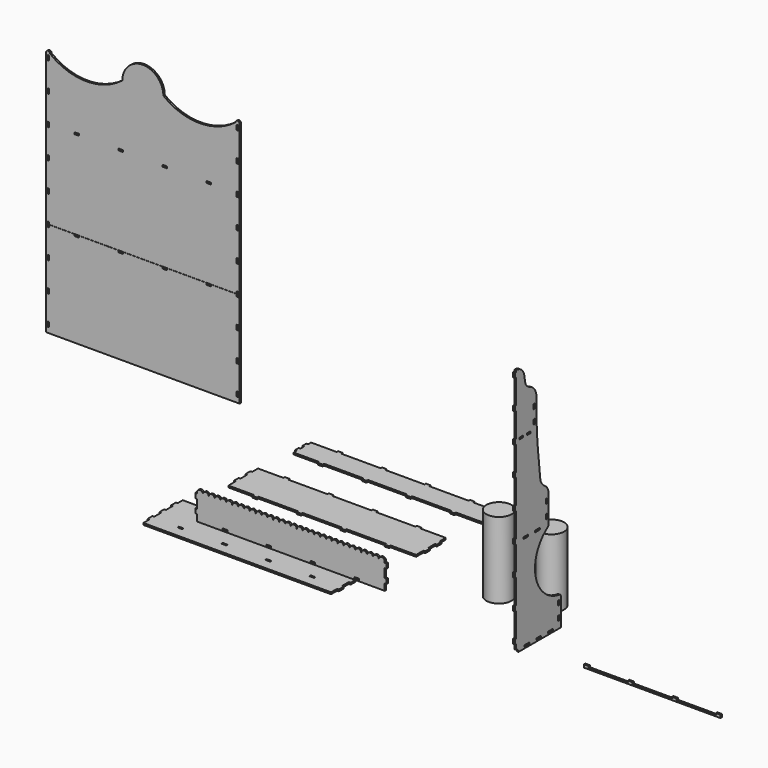
from build123d import *

# Parameters (mm, degrees)
F0_W      = 10
F0_H      = 3
F0_W_2    = 3
F0_H_2    = 8
F0_W_3    = 8
F1_DEPTH  = 3
F2_W      = 8
F2_H      = 3
F3_DEPTH  = 3
F4_W      = 8
F4_H      = 3
F5_DEPTH  = 3
F7_DEPTH  = 3
F9_DEPTH  = 3
F10_W     = 3
F10_H     = 8
F12_DEPTH = 3
F10_W_2   = 8
F10_H_2   = 3
F13_DEPTH = 3
F14_DEPTH = 3
F15_R     = 21.5
F16_DEPTH = 130
F17_DEPTH = 117


# Not quite as in the source:
# - a feature names something its author has since deleted; it is built from what else it names


with BuildPart() as f1:
    # F0 (on Right) → F1 (new body)
    with BuildSketch(Plane.YZ):
        with BuildLine():
            Line((0, 14), (0, 5))
            ThreePointArc((0, 5), (3.5355339059, 3.5355339059), (5, 0))
            Line((5, 0), (95, 0))
            Line((95, 0), (95, 47.3543956658))
            ThreePointArc((95, 47.3543956658), (94.2705921351, 49.3151127173), (92.4370590961, 50.3223881433))
            ThreePointArc((92.4370590961, 50.3223881433), (41.6413829378, 97.2032586539), (66.8184709068, 161.5781837226))
            ThreePointArc((66.8184709068, 161.5781837226), (68.4211058873, 163.372759507), (69, 165.7081016089))
            Line((69, 165.7081016089), (69, 213))
            ThreePointArc((69, 213), (66.3858613305, 220.9035210379), (60.5112875599, 226.8017198134))
            ThreePointArc((60.5112875599, 226.8017198134), (54.1229379519, 233.1545161459), (51.1709644901, 241.6665596512))
            Line((51.1709644901, 241.6665596512), (46.9762373129, 280.85384986))
            ThreePointArc((46.9762373129, 280.85384986), (45.2396853535, 299.4070999888), (43.9976015301, 318))
            ThreePointArc((43.9976015301, 318), (43.2494448273, 336.6725204464), (43, 355.3583582802))
            Line((43, 355.3583582802), (43, 369.5985722542))
            ThreePointArc((43, 369.5985722542), (38.5808045495, 380.9800883223), (28.6916338415, 388.1405700899))
            ThreePointArc((28.6916338415, 388.1405700899), (22.2280112249, 392.6087038732), (18.9101247071, 399.7315028939))
            Line((18.9101247071, 399.7315028939), (17.4928194431, 407.943180155))
            ThreePointArc((17.4928194431, 407.943180155), (12.2161147188, 420.0299862844), (0, 425))
            Line((0, 425), (0, 422))
            Line((0, 422), (-3, 422))
            Line((-3, 422), (-3, 414))
            Line((-3, 414), (0, 414))
            Line((0, 414), (0, 372))
            Line((0, 372), (-3, 372))
            Line((-3, 372), (-3, 364))
            Line((-3, 364), (0, 364))
            Line((0, 364), (0, 322))
            Line((0, 322), (-3, 322))
            Line((-3, 322), (-3, 314))
            Line((-3, 314), (0, 314))
            Line((0, 314), (0, 272))
            Line((0, 272), (-3, 272))
            Line((-3, 272), (-3, 264))
            Line((-3, 264), (0, 264))
            Line((0, 264), (0, 222))
            Line((0, 222), (-3, 222))
            Line((-3, 222), (-3, 214))
            Line((-3, 214), (0, 214))
            Line((0, 214), (0, 172))
            Line((0, 172), (-3, 172))
            Line((-3, 172), (-3, 164))
            Line((-3, 164), (0, 164))
            Line((0, 164), (0, 122))
            Line((0, 122), (-3, 122))
            Line((-3, 122), (-3, 114))
            Line((-3, 114), (0, 114))
            Line((0, 114), (0, 72))
            Line((0, 72), (-3, 72))
            Line((-3, 72), (-3, 64))
            Line((-3, 64), (0, 64))
            Line((0, 64), (0, 22))
            Line((0, 22), (-3, 22))
            Line((-3, 22), (-3, 14))
            Line((-3, 14), (0, 14))
        make_face()
        with Locations((23, 3.5)):
            Rectangle(F0_W, F0_H, mode=Mode.SUBTRACT)
        with Locations((20.5, 166.5)):
            Rectangle(F0_W, F0_H, mode=Mode.SUBTRACT)
        with Locations((45.5, 166.5)):
            Rectangle(F0_W, F0_H, mode=Mode.SUBTRACT)
        with Locations((48, 3.5)):
            Rectangle(F0_W, F0_H, mode=Mode.SUBTRACT)
        with Locations((73, 3.5)):
            Rectangle(F0_W, F0_H, mode=Mode.SUBTRACT)
        with Locations((90.5, 16)):
            Rectangle(F0_W_2, F0_H_2, mode=Mode.SUBTRACT)
        with Locations((90.5, 39)):
            Rectangle(F0_W_2, F0_H_2, mode=Mode.SUBTRACT)
        with Locations((64.5, 179)):
            Rectangle(F0_W_2, F0_H_2, mode=Mode.SUBTRACT)
        with Locations((64.5, 202)):
            Rectangle(F0_W_2, F0_H_2, mode=Mode.SUBTRACT)
        with Locations((10.5, 319.5)):
            Rectangle(F0_W_3, F0_H, mode=Mode.SUBTRACT)
        with Locations((26.5, 319.5)):
            Rectangle(F0_W_3, F0_H, mode=Mode.SUBTRACT)
        with Locations((38.5, 332)):
            Rectangle(F0_W_2, F0_H_2, mode=Mode.SUBTRACT)
        with Locations((38.5, 355)):
            Rectangle(F0_W_2, F0_H_2, mode=Mode.SUBTRACT)
    extrude(amount=F1_DEPTH)


with BuildPart() as f3:
    # F2 (on Top) → F3 (new body)
    with BuildSketch(Plane.XY):
        Polygon((-615.7709360123, -8.2306790054), (-615.7709360123, -21.2306790054), (-295.7709360123, -21.2306790054), (-295.7709360123, -8.2306790054), (-292.7709360123, -8.2306790054), (-292.7709360123, 1.7693209946), (-295.7709360123, 1.7693209946), (-295.7709360123, 16.7693209946), (-292.7709360123, 16.7693209946), (-292.7709360123, 26.7693209946), (-295.7709360123, 26.7693209946), (-295.7709360123, 41.7693209946), (-292.7709360123, 41.7693209946), (-292.7709360123, 51.7693209946), (-295.7709360123, 51.7693209946), (-295.7709360123, 62.7693209946), (-339.2709360123, 62.7693209946), (-339.2709360123, 65.7693209946), (-347.2709360123, 65.7693209946), (-347.2709360123, 62.7693209946), (-414.2709360123, 62.7693209946), (-414.2709360123, 65.7693209946), (-422.2709360123, 65.7693209946), (-422.2709360123, 62.7693209946), (-489.2709360123, 62.7693209946), (-489.2709360123, 65.7693209946), (-497.2709360123, 65.7693209946), (-497.2709360123, 62.7693209946), (-564.2709360123, 62.7693209946), (-564.2709360123, 65.7693209946), (-572.2709360123, 65.7693209946), (-572.2709360123, 62.7693209946), (-615.7709360123, 62.7693209946), (-615.7709360123, 51.7693209946), (-618.7709360123, 51.7693209946), (-618.7709360123, 41.7693209946), (-615.7709360123, 41.7693209946), (-615.7709360123, 26.7693209946), (-618.7709360123, 26.7693209946), (-618.7709360123, 16.7693209946), (-615.7709360123, 16.7693209946), (-615.7709360123, 1.7693209946), (-618.7709360123, 1.7693209946), (-618.7709360123, -8.2306790054), align=None)
        with Locations((-568.2709360123, -1.5)):
            Rectangle(F2_W, F2_H, mode=Mode.SUBTRACT)
        with Locations((-493.2709360123, -1.5)):
            Rectangle(F2_W, F2_H, mode=Mode.SUBTRACT)
        with Locations((-418.2709360123, -1.5)):
            Rectangle(F2_W, F2_H, mode=Mode.SUBTRACT)
        with Locations((-343.2709360123, -1.5)):
            Rectangle(F2_W, F2_H, mode=Mode.SUBTRACT)
    extrude(amount=F3_DEPTH)


with BuildPart() as f5:
    # F4 (on Front) → F5 (new body)
    with BuildSketch(Plane.XZ):
        with BuildLine():
            Line((-538.8287305832, 22.7397029996), (-218.8287305832, 22.7397029996))
            Line((-218.8287305832, 22.7397029996), (-218.8287305832, 33.7397029996))
            Line((-218.8287305832, 33.7397029996), (-215.8287305832, 33.7397029996))
            Line((-215.8287305832, 33.7397029996), (-215.8287305832, 41.7397029996))
            Line((-215.8287305832, 41.7397029996), (-218.8287305832, 41.7397029996))
            Line((-218.8287305832, 41.7397029996), (-218.8287305832, 56.7397029996))
            Line((-218.8287305832, 56.7397029996), (-215.8287305832, 56.7397029996))
            Line((-215.8287305832, 56.7397029996), (-215.8287305832, 64.7397029996))
            Line((-215.8287305832, 64.7397029996), (-218.8287305832, 64.7397029996))
            Line((-218.8287305832, 64.7397029996), (-218.8287305832, 66.7397029996))
            ThreePointArc((-218.8287305832, 66.7397029996), (-223.8287305832, 71.7397029996), (-228.8287305832, 66.7397029996))
            ThreePointArc((-228.8287305832, 66.7397029996), (-233.8287305832, 71.7397029996), (-238.8287305832, 66.7397029996))
            ThreePointArc((-238.8287305832, 66.7397029996), (-243.8287305832, 71.7397029996), (-248.8287305832, 66.7397029996))
            ThreePointArc((-248.8287305832, 66.7397029996), (-253.8287305832, 71.7397029996), (-258.8287305832, 66.7397029996))
            ThreePointArc((-258.8287305832, 66.7397029996), (-263.8287305832, 71.7397029996), (-268.8287305832, 66.7397029996))
            ThreePointArc((-268.8287305832, 66.7397029996), (-273.8287305832, 71.7397029996), (-278.8287305832, 66.7397029996))
            ThreePointArc((-278.8287305832, 66.7397029996), (-283.8287305832, 71.7397029996), (-288.8287305832, 66.7397029996))
            ThreePointArc((-288.8287305832, 66.7397029996), (-293.8287305832, 71.7397029996), (-298.8287305832, 66.7397029996))
            ThreePointArc((-298.8287305832, 66.7397029996), (-303.8287305832, 71.7397029996), (-308.8287305832, 66.7397029996))
            ThreePointArc((-308.8287305832, 66.7397029996), (-313.8287305832, 71.7397029996), (-318.8287305832, 66.7397029996))
            ThreePointArc((-318.8287305832, 66.7397029996), (-323.8287305832, 71.7397029996), (-328.8287305832, 66.7397029996))
            ThreePointArc((-328.8287305832, 66.7397029996), (-333.8287305832, 71.7397029996), (-338.8287305832, 66.7397029996))
            ThreePointArc((-338.8287305832, 66.7397029996), (-343.8287305832, 71.7397029996), (-348.8287305832, 66.7397029996))
            ThreePointArc((-348.8287305832, 66.7397029996), (-353.8287305832, 71.7397029996), (-358.8287305832, 66.7397029996))
            ThreePointArc((-358.8287305832, 66.7397029996), (-363.8287305832, 71.7397029996), (-368.8287305832, 66.7397029996))
            ThreePointArc((-368.8287305832, 66.7397029996), (-373.8287305832, 71.7397029996), (-378.8287305832, 66.7397029996))
            ThreePointArc((-378.8287305832, 66.7397029996), (-383.8287305832, 71.7397029996), (-388.8287305832, 66.7397029996))
            ThreePointArc((-388.8287305832, 66.7397029996), (-393.8287305832, 71.7397029996), (-398.8287305832, 66.7397029996))
            ThreePointArc((-398.8287305832, 66.7397029996), (-403.8287305832, 71.7397029996), (-408.8287305832, 66.7397029996))
            ThreePointArc((-408.8287305832, 66.7397029996), (-413.8287305832, 71.7397029996), (-418.8287305832, 66.7397029996))
            ThreePointArc((-418.8287305832, 66.7397029996), (-423.8287305832, 71.7397029996), (-428.8287305832, 66.7397029996))
            ThreePointArc((-428.8287305832, 66.7397029996), (-433.8287305832, 71.7397029996), (-438.8287305832, 66.7397029996))
            ThreePointArc((-438.8287305832, 66.7397029996), (-443.8287305832, 71.7397029996), (-448.8287305832, 66.7397029996))
            ThreePointArc((-448.8287305832, 66.7397029996), (-453.8287305832, 71.7397029996), (-458.8287305832, 66.7397029996))
            ThreePointArc((-458.8287305832, 66.7397029996), (-463.8287305832, 71.7397029996), (-468.8287305832, 66.7397029996))
            ThreePointArc((-468.8287305832, 66.7397029996), (-473.8287305832, 71.7397029996), (-478.8287305832, 66.7397029996))
            ThreePointArc((-478.8287305832, 66.7397029996), (-483.8287305832, 71.7397029996), (-488.8287305832, 66.7397029996))
            ThreePointArc((-488.8287305832, 66.7397029996), (-493.8287305832, 71.7397029996), (-498.8287305832, 66.7397029996))
            ThreePointArc((-498.8287305832, 66.7397029996), (-503.8287305832, 71.7397029996), (-508.8287305832, 66.7397029996))
            ThreePointArc((-508.8287305832, 66.7397029996), (-513.8287305832, 71.7397029996), (-518.8287305832, 66.7397029996))
            ThreePointArc((-518.8287305832, 66.7397029996), (-523.8287305832, 71.7397029996), (-528.8287305832, 66.7397029996))
            ThreePointArc((-528.8287305832, 66.7397029996), (-533.8287305832, 71.7397029996), (-538.8287305832, 66.7397029996))
            Line((-538.8287305832, 66.7397029996), (-538.8287305832, 64.7397029996))
            Line((-538.8287305832, 64.7397029996), (-541.8287305832, 64.7397029996))
            Line((-541.8287305832, 64.7397029996), (-541.8287305832, 56.7397029996))
            Line((-541.8287305832, 56.7397029996), (-538.8287305832, 56.7397029996))
            Line((-538.8287305832, 56.7397029996), (-538.8287305832, 41.7397029996))
            Line((-538.8287305832, 41.7397029996), (-541.8287305832, 41.7397029996))
            Line((-541.8287305832, 41.7397029996), (-541.8287305832, 33.7397029996))
            Line((-541.8287305832, 33.7397029996), (-538.8287305832, 33.7397029996))
            Line((-538.8287305832, 33.7397029996), (-538.8287305832, 22.7397029996))
        make_face()
        with Locations((-491.3287305832, 25.2397029996)):
            Rectangle(F4_W, F4_H, mode=Mode.SUBTRACT)
        with Locations((-416.3287305832, 25.2397029996)):
            Rectangle(F4_W, F4_H, mode=Mode.SUBTRACT)
        with Locations((-341.3287305832, 25.2397029996)):
            Rectangle(F4_W, F4_H, mode=Mode.SUBTRACT)
        with Locations((-266.3287305832, 25.2397029996)):
            Rectangle(F4_W, F4_H, mode=Mode.SUBTRACT)
    extrude(amount=F5_DEPTH)


with BuildPart() as f7:
    # F6 (on Top) → F7 (new body)
    with BuildSketch(Plane.XY):
        Polygon((-551.2527956963, 196.7857158184), (-594.7527956963, 196.7857158184), (-594.7527956963, 184.2857158184), (-597.7527956963, 184.2857158184), (-597.7527956963, 174.2857158184), (-594.7527956963, 174.2857158184), (-594.7527956963, 159.2857158184), (-597.7527956963, 159.2857158184), (-597.7527956963, 149.2857158184), (-594.7527956963, 149.2857158184), (-594.7527956963, 133.7857158184), (-551.2527956963, 133.7857158184), (-551.2527956963, 130.7857158184), (-543.2527956963, 130.7857158184), (-543.2527956963, 133.7857158184), (-476.2527956963, 133.7857158184), (-476.2527956963, 130.7857158184), (-468.2527956963, 130.7857158184), (-468.2527956963, 133.7857158184), (-401.2527956963, 133.7857158184), (-401.2527956963, 130.7857158184), (-393.2527956963, 130.7857158184), (-393.2527956963, 133.7857158184), (-326.2527956963, 133.7857158184), (-326.2527956963, 130.7857158184), (-318.2527956963, 130.7857158184), (-318.2527956963, 133.7857158184), (-274.7527956963, 133.7857158184), (-274.7527956963, 149.2857158184), (-271.7527956963, 149.2857158184), (-271.7527956963, 159.2857158184), (-274.7527956963, 159.2857158184), (-274.7527956963, 174.2857158184), (-271.7527956963, 174.2857158184), (-271.7527956963, 184.2857158184), (-274.7527956963, 184.2857158184), (-274.7527956963, 196.7857158184), (-318.2527956963, 196.7857158184), (-318.2527956963, 199.7857158184), (-326.2527956963, 199.7857158184), (-326.2527956963, 196.7857158184), (-393.2527956963, 196.7857158184), (-393.2527956963, 199.7857158184), (-401.2527956963, 199.7857158184), (-401.2527956963, 196.7857158184), (-468.2527956963, 196.7857158184), (-468.2527956963, 199.7857158184), (-476.2527956963, 199.7857158184), (-476.2527956963, 196.7857158184), (-543.2527956963, 196.7857158184), (-543.2527956963, 199.7857158184), (-551.2527956963, 199.7857158184), align=None)
    extrude(amount=F7_DEPTH)


with BuildPart() as f9:
    # F8 (on Top) → F9 (new body)
    with BuildSketch(Plane.XY):
        Polygon((-542.8163928986, 299.3931765556), (-586.3163928986, 299.3931765556), (-586.3163928986, 292.8931765556), (-589.3163928986, 292.8931765556), (-589.3163928986, 284.8931765556), (-586.3163928986, 284.8931765556), (-586.3163928986, 276.8931765556), (-589.3163928986, 276.8931765556), (-589.3163928986, 268.8931765556), (-586.3163928986, 268.8931765556), (-586.3163928986, 262.3931765556), (-542.8163928986, 262.3931765556), (-542.8163928986, 259.3931765556), (-534.8163928986, 259.3931765556), (-534.8163928986, 262.3931765556), (-467.8163928986, 262.3931765556), (-467.8163928986, 259.3931765556), (-459.8163928986, 259.3931765556), (-459.8163928986, 262.3931765556), (-392.8163928986, 262.3931765556), (-392.8163928986, 259.3931765556), (-384.8163928986, 259.3931765556), (-384.8163928986, 262.3931765556), (-317.8163928986, 262.3931765556), (-317.8163928986, 259.3931765556), (-309.8163928986, 259.3931765556), (-309.8163928986, 262.3931765556), (-266.3163928986, 262.3931765556), (-266.3163928986, 268.8931765556), (-263.3163928986, 268.8931765556), (-263.3163928986, 276.8931765556), (-266.3163928986, 276.8931765556), (-266.3163928986, 284.8931765556), (-263.3163928986, 284.8931765556), (-263.3163928986, 292.8931765556), (-266.3163928986, 292.8931765556), (-266.3163928986, 299.3931765556), (-309.8163928986, 299.3931765556), (-309.8163928986, 302.3931765556), (-317.8163928986, 302.3931765556), (-317.8163928986, 299.3931765556), (-384.8163928986, 299.3931765556), (-384.8163928986, 302.3931765556), (-392.8163928986, 302.3931765556), (-392.8163928986, 299.3931765556), (-459.8163928986, 299.3931765556), (-459.8163928986, 302.3931765556), (-467.8163928986, 302.3931765556), (-467.8163928986, 299.3931765556), (-534.8163928986, 299.3931765556), (-534.8163928986, 302.3931765556), (-542.8163928986, 302.3931765556), align=None)
    extrude(amount=F9_DEPTH)


with BuildPart() as f12:
    # F10 (on Front) → F12 (new body)
    with BuildSketch(Plane.XZ):
        Polygon((-796.2708473206, 223.258972168), (-466.2708473206, 223.258972168), (-466.2708473206, 386.258972168), (-468.2708473206, 386.258972168), (-468.2708473206, 382.258972168), (-471.2708473206, 382.258972168), (-471.2708473206, 386.258972168), (-514.7708473206, 386.258972168), (-514.7708473206, 383.258972168), (-522.7708473206, 383.258972168), (-522.7708473206, 386.258972168), (-589.7708473206, 386.258972168), (-589.7708473206, 383.258972168), (-597.7708473206, 383.258972168), (-597.7708473206, 386.258972168), (-664.7708473206, 386.258972168), (-664.7708473206, 383.258972168), (-672.7708473206, 383.258972168), (-672.7708473206, 386.258972168), (-739.7708473206, 386.258972168), (-739.7708473206, 383.258972168), (-747.7708473206, 383.258972168), (-747.7708473206, 386.258972168), (-791.2708473206, 386.258972168), (-791.2708473206, 382.258972168), (-794.2708473206, 382.258972168), (-794.2708473206, 386.258972168), (-796.2708473206, 386.258972168), align=None)
        with Locations((-792.7708473206, 236.258972168)):
            Rectangle(F10_W, F10_H, mode=Mode.SUBTRACT)
        with Locations((-792.7708473206, 286.258972168)):
            Rectangle(F10_W, F10_H, mode=Mode.SUBTRACT)
        with Locations((-792.7708473206, 336.258972168)):
            Rectangle(F10_W, F10_H, mode=Mode.SUBTRACT)
        with Locations((-469.7708473206, 236.258972168)):
            Rectangle(F10_W, F10_H, mode=Mode.SUBTRACT)
        with Locations((-469.7708473206, 286.258972168)):
            Rectangle(F10_W, F10_H, mode=Mode.SUBTRACT)
        with Locations((-469.7708473206, 336.258972168)):
            Rectangle(F10_W, F10_H, mode=Mode.SUBTRACT)
    extrude(amount=F12_DEPTH)


with BuildPart() as f13:
    # F10 (on Front) → F13 (new body)
    with BuildSketch(Plane.XZ):
        with BuildLine():
            ThreePointArc((-473.2708473206, 643.258972168), (-534.7708473206, 622.1116829647), (-596.2708473206, 643.258972168))
            ThreePointArc((-596.2708473206, 643.258972168), (-631.2708473206, 678.258972168), (-666.2708473206, 643.258972168))
            ThreePointArc((-666.2708473206, 643.258972168), (-727.7708473206, 622.1116829647), (-789.2708473206, 643.258972168))
            ThreePointArc((-789.2708473206, 643.258972168), (-792.7708473206, 646.758972168), (-796.2708473206, 643.258972168))
            Line((-796.2708473206, 643.258972168), (-796.2708473206, 386.458972168))
            Line((-796.2708473206, 386.458972168), (-794.2708473206, 386.458972168))
            Line((-794.2708473206, 386.458972168), (-794.2708473206, 390.258972168))
            Line((-794.2708473206, 390.258972168), (-791.2708473206, 390.258972168))
            Line((-791.2708473206, 390.258972168), (-791.2708473206, 386.458972168))
            Line((-791.2708473206, 386.458972168), (-471.2708473206, 386.458972168))
            Line((-471.2708473206, 386.458972168), (-471.2708473206, 390.258972168))
            Line((-471.2708473206, 390.258972168), (-468.2708473206, 390.258972168))
            Line((-468.2708473206, 390.258972168), (-468.2708473206, 386.458972168))
            Line((-468.2708473206, 386.458972168), (-466.2708473206, 386.458972168))
            Line((-466.2708473206, 386.458972168), (-466.2708473206, 643.258972168))
            ThreePointArc((-466.2708473206, 643.258972168), (-469.7708473206, 646.758972168), (-473.2708473206, 643.258972168))
        make_face()
        with Locations((-792.7708473206, 436.258972168)):
            Rectangle(F10_W, F10_H, mode=Mode.SUBTRACT)
        with Locations((-469.7708473206, 436.258972168)):
            Rectangle(F10_W, F10_H, mode=Mode.SUBTRACT)
        with Locations((-792.7708473206, 486.258972168)):
            Rectangle(F10_W, F10_H, mode=Mode.SUBTRACT)
        with Locations((-792.7708473206, 536.258972168)):
            Rectangle(F10_W, F10_H, mode=Mode.SUBTRACT)
        with Locations((-743.7708473206, 537.758972168)):
            Rectangle(F10_W_2, F10_H_2, mode=Mode.SUBTRACT)
        with Locations((-668.7708473206, 537.758972168)):
            Rectangle(F10_W_2, F10_H_2, mode=Mode.SUBTRACT)
        with Locations((-792.7708473206, 586.258972168)):
            Rectangle(F10_W, F10_H, mode=Mode.SUBTRACT)
        with Locations((-792.7708473206, 636.258972168)):
            Rectangle(F10_W, F10_H, mode=Mode.SUBTRACT)
        with Locations((-593.7708473206, 537.758972168)):
            Rectangle(F10_W_2, F10_H_2, mode=Mode.SUBTRACT)
        with Locations((-518.7708473206, 537.758972168)):
            Rectangle(F10_W_2, F10_H_2, mode=Mode.SUBTRACT)
        with Locations((-469.7708473206, 486.258972168)):
            Rectangle(F10_W, F10_H, mode=Mode.SUBTRACT)
        with Locations((-469.7708473206, 536.258972168)):
            Rectangle(F10_W, F10_H, mode=Mode.SUBTRACT)
        with Locations((-469.7708473206, 586.258972168)):
            Rectangle(F10_W, F10_H, mode=Mode.SUBTRACT)
        with Locations((-469.7708473206, 636.258972168)):
            Rectangle(F10_W, F10_H, mode=Mode.SUBTRACT)
    extrude(amount=F13_DEPTH)


with BuildPart() as f14:
    # F11 (on Front) → F14 (new body)
    with BuildSketch(Plane.XZ):
        Polygon((128.7609785795, 22.9280899465), (120.7609785795, 22.9280899465), (120.7609785795, 17.9280899465), (128.7609785795, 17.9280899465), (195.7609785795, 17.9280899465), (203.7609785795, 17.9280899465), (270.7609785795, 17.9280899465), (278.7609785795, 17.9280899465), (345.7609785795, 17.9280899465), (353.7609785795, 17.9280899465), (353.7609785795, 22.9280899465), (345.7609785795, 22.9280899465), (345.7609785795, 19.9280899465), (278.7609785795, 19.9280899465), (278.7609785795, 22.9280899465), (270.7609785795, 22.9280899465), (270.7609785795, 19.9280899465), (203.7609785795, 19.9280899465), (203.7609785795, 22.9280899465), (195.7609785795, 22.9280899465), (195.7609785795, 19.9280899465), (128.7609785795, 19.9280899465), align=None)
    extrude(amount=F14_DEPTH)


with BuildPart() as f16:
    # F15 (on Top) → F16 (new body)
    with BuildSketch(Plane.XY):
        with Locations((-117.7703887224, 114.1628473997)):
            Circle(F15_R)
    extrude(amount=F16_DEPTH)


with BuildPart() as f17:
    # F15 (on Top) → F17 (new body)
    with BuildSketch(Plane.XY):
        with Locations((-47.3840460181, 138.1680816412)):
            Circle(F15_R)
    extrude(amount=F17_DEPTH)


solid = Compound([f1.part, f3.part, f5.part, f7.part, f9.part, f12.part, f13.part, f14.part, f16.part, f17.part])
